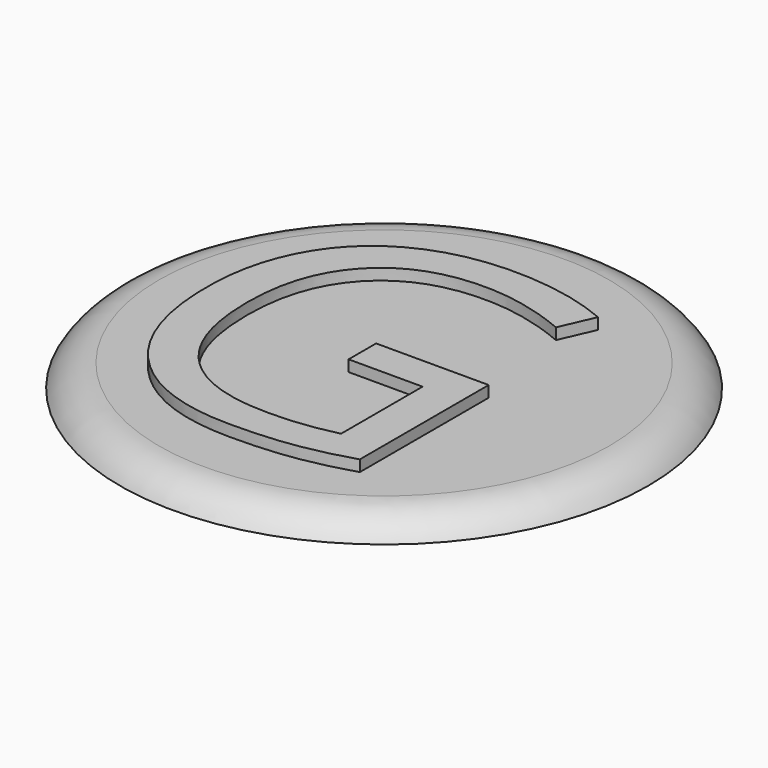
from build123d import *

# Parameters (mm, degrees)
F0_R         = 11.75
F1_DEPTH     = 1
F2_TEXT_SIZE = 20.6489181936
F3_DEPTH     = 0.5


# Not quite as in the source:
# - a fillet or chamfer that OpenCascade refuses, or shapes differently, is made with other operations: its cross-section is extruded or revolved along the edge and cut away or added
# - Text() gives the source's letters only with a copy of the font that has no kerning and outlines rounded to 1/6400 em; it was checked with that copy


with BuildPart() as f1:
    # F0 (on Top) → F1 (new body)
    with BuildSketch(Plane.XY):
        Circle(F0_R)
    extrude(amount=F1_DEPTH)

    # F2 (on face) → F3 (join)
    with BuildSketch(Plane.XY.offset(1)):
        with Locations((-9.0446764926, -7.5004217977)):
            Text('G', F2_TEXT_SIZE, font='Open Sans', text_align=(TextAlign.LEFT, TextAlign.BOTTOM))
    extrude(amount=F3_DEPTH)

    # F4: fillet of radius 2 on 1 edges, made by hand

    # F4_s1 → F4_t2 (revolve, cut)
    with BuildSketch(Plane.XZ):
        with BuildLine():
            ThreePointArc((11.75, 0), (11.0179491924, 0.7320508076), (10.0179491924, 1))
            Line((10.0179491924, 1), (11.75, 1))
            Line((11.75, 1), (11.75, 0))
        make_face()
    revolve(axis=Axis((0, 0, 1), (0, 0, 1)), mode=Mode.SUBTRACT)


solid = f1.part
